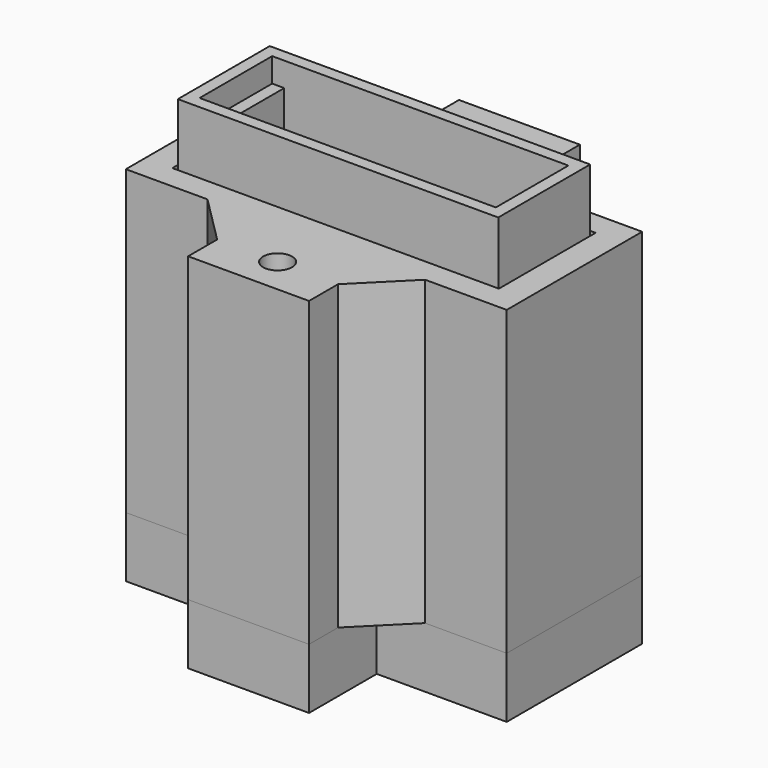
from build123d import *

# Parameters (mm, degrees)
F0_W      = 26.5
F0_H      = 9.5
F1_DEPTH  = 13
F2_W      = 26.5
F2_H      = 9.5
F2_W_2    = 24.5
F2_H_2    = 7.5
F3_DEPTH  = 6
F4_W      = 1
F4_H      = 7.5
F5_DEPTH  = 4
F6_R      = 3.1
F7_DEPTH  = 19
F8_W      = 1.5
F8_H      = 9.5
F9_DEPTH  = 9
F10_R     = 2.55
F11_DEPTH = 3
F13_W     = 27
F13_H     = 10
F13_W_2   = 10
F13_H_2   = 7
F14_DEPTH = 25
F15_W     = 30
F15_H     = 10
F16_DEPTH = 20
F17_R     = 1.2
F18_DEPTH = 25
F19_W     = 5
F19_H     = 5
F19_R     = 4
F19_W_2   = 10
F19_H_2   = 7
F19_R_2   = 1.5
F20_DEPTH = 5
F21_SIZE  = 4
F23_W     = 5
F23_H     = 9
F24_DEPTH = 11


with BuildPart() as f1:
    # F0 (on Top) → F1 (new body)
    with BuildSketch(Plane.XY):
        Rectangle(F0_W, F0_H)
    extrude(amount=F1_DEPTH)

    # F2 (on face) → F3 (join)
    with BuildSketch(Plane.XY.offset(13)):
        Rectangle(F2_W, F2_H)
        Rectangle(F2_W_2, F2_H_2, mode=Mode.SUBTRACT)
    extrude(amount=F3_DEPTH)

    # F4 (on face) → F5 (join)
    with BuildSketch(Plane.XY.offset(13)):
        with Locations((-11.75, 0)):
            Rectangle(F4_W, F4_H)
        with Locations((11.75, 0)):
            Rectangle(F4_W, F4_H)
    extrude(amount=F5_DEPTH)

    # F6 (on face) → F7 (cut)
    with BuildSketch(Plane.XY.offset(13)):
        with Locations((-6.5, 0)):
            Circle(F6_R)
        with Locations((6.5, 0)):
            Circle(F6_R)
    extrude(amount=-F7_DEPTH, mode=Mode.SUBTRACT)

    # F8 (on face) → F9 (join)
    with BuildSketch(Plane(origin=(0, 0, 0), x_dir=(1, 0, 0), z_dir=(0, 0, -1))):
        with Locations((-14, 0)):
            Rectangle(F8_W, F8_H)
        with Locations((14, 0)):
            Rectangle(F8_W, F8_H)
    extrude(amount=-F9_DEPTH)

    # F10 (on face) → F11 (cut)
    with BuildSketch(Plane(origin=(0, 0, 0), x_dir=(1, 0, 0), z_dir=(0, 0, -1))):
        Circle(F10_R)
    extrude(amount=-F11_DEPTH, mode=Mode.SUBTRACT)


with BuildPart() as f14:
    # F13 (on offset) → F14 (new body)
    with BuildSketch(Plane.XY.offset(14)):
        Polygon((5, -7), (15.75, -7), (15.75, 7), (5, 7), (-5, 7), (-15.75, 7), (-15.75, -7), (-5, -7), align=None)
        Rectangle(F13_W, F13_H, mode=Mode.SUBTRACT)
        with Locations((0, -10.5)):
            Rectangle(F13_W_2, F13_H_2)
        with Locations((0, 10.5)):
            Rectangle(F13_W_2, F13_H_2)
    extrude(amount=-F14_DEPTH)

    # F15 (on face) → F16 (cut)
    with BuildSketch(Plane(origin=(0, 0, -11), x_dir=(1, 0, 0), z_dir=(0, 0, -1))):
        Rectangle(F15_W, F15_H)
    extrude(amount=-F16_DEPTH, mode=Mode.SUBTRACT)

    # F17 (on face) → F18 (cut)
    with BuildSketch(Plane.XY.offset(14)):
        with Locations((0, 11)):
            Circle(F17_R)
        with Locations((0, -11)):
            Circle(F17_R)
    extrude(amount=-F18_DEPTH, mode=Mode.SUBTRACT)

    # F21
    f21_edges = [f14.edges().sort_by_distance(p)[0] for p in [
        (-5, 7, 1.5),
        (5, 7, 1.5),
        (5, -7, 1.5),
        (-5, -7, 1.5),
    ]]
    chamfer(f21_edges, length=F21_SIZE)


with BuildPart() as f20:
    # F19 (on face) → F20 (new body)
    with BuildSketch(Plane(origin=(0, 0, -11), x_dir=(1, 0, 0), z_dir=(0, 0, -1))):
        Polygon((5, -7), (15.75, -7), (15.75, 7), (5, 7), (-5, 7), (-15.75, 7), (-15.75, -7), (-5, -7), align=None)
        with Locations((-7.5, 0)):
            Rectangle(F19_W, F19_H, mode=Mode.SUBTRACT)
        Circle(F19_R, mode=Mode.SUBTRACT)
        with Locations((7.5, 0)):
            Rectangle(F19_W, F19_H, mode=Mode.SUBTRACT)
        with Locations((0, -10.5)):
            Rectangle(F19_W_2, F19_H_2)
        with Locations((0, -11)):
            Circle(F19_R_2, mode=Mode.SUBTRACT)
        with Locations((0, 10.5)):
            Rectangle(F19_W_2, F19_H_2)
        with Locations((0, 11)):
            Circle(F19_R_2, mode=Mode.SUBTRACT)
    extrude(amount=F20_DEPTH)


with BuildPart() as f24:
    # F23 (on offset) → F24 (new body)
    with BuildSketch(Plane(origin=(0, 0, -11), x_dir=(1, 0, 0), z_dir=(0, 0, -1))):
        Rectangle(F23_W, F23_H)
    extrude(amount=-F24_DEPTH)


solid = Compound([f1.part, f14.part, f20.part, f24.part])
